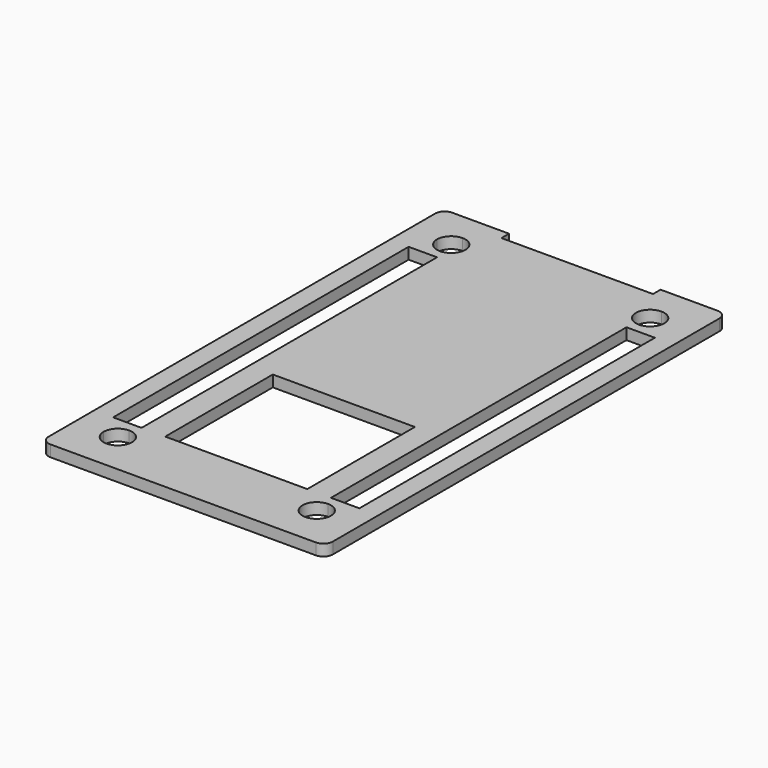
from build123d import *

# Parameters (mm, degrees)
F0_W     = 4
F0_H     = 1
F0_W_2   = 2
F0_H_2   = 39
F0_W_3   = 2.5
F0_H_3   = 0.8
F0_W_4   = 7.5
F0_W_5   = 0.5
F1_DEPTH = 1.2


with BuildPart() as f1:
    # F0 (on Top) → F1 (new body)
    with BuildSketch(Plane.XY):
        with BuildLine():
            Line((-13, 24.5), (-12, 24.5))
            Line((-12, 24.5), (-10.5, 24.5))
            Line((-10.5, 24.5), (-8, 24.5))
            Line((-8, 24.5), (-8, 25.5))
            Line((-8, 25.5), (-8, 26.5))
            Line((-8, 26.5), (-14, 26.5))
            ThreePointArc((-14, 26.5), (-14.7071067812, 26.2071067812), (-15, 25.5))
            Line((-15, 25.5), (-15, 19.5))
            Line((-15, 19.5), (-13, 19.5))
            Line((-13, 19.5), (-13, 22))
            Line((-13, 22), (-13, 23.5))
            Line((-13, 23.5), (-13, 24.5))
        make_face()
        with BuildLine():
            Line((-10.5, 24.5), (-12, 24.5))
            ThreePointArc((-12, 24.5), (-12.7071067812, 24.2071067812), (-13, 23.5))
            Line((-13, 23.5), (-13, 22))
            Line((-13, 22), (-12, 22))
            ThreePointArc((-12, 22), (-11.5606601718, 23.0606601718), (-10.5, 23.5))
            Line((-10.5, 23.5), (-10.5, 24.5))
        make_face()
        with BuildLine():
            ThreePointArc((-13, 23.5), (-12.7071067812, 24.2071067812), (-12, 24.5))
            Line((-12, 24.5), (-13, 24.5))
            Line((-13, 24.5), (-13, 23.5))
        make_face()
        with BuildLine():
            Line((-8, 24.5), (-10.5, 24.5))
            Line((-10.5, 24.5), (-10.5, 23.5))
            ThreePointArc((-10.5, 23.5), (-9.4393398282, 23.0606601718), (-9, 22))
            ThreePointArc((-9, 22), (-9.4393398282, 20.9393398282), (-10.5, 20.5))
            Line((-10.5, 20.5), (-10.5, 19.5))
            Line((-10.5, 19.5), (-10, 19.5))
            Line((-10, 19.5), (10, 19.5))
            Line((10, 19.5), (10.5, 19.5))
            Line((10.5, 19.5), (10.5, 20.5))
            ThreePointArc((10.5, 20.5), (9, 22), (10.5, 23.5))
            Line((10.5, 23.5), (10.5, 24.5))
            Line((10.5, 24.5), (8, 24.5))
            Line((8, 24.5), (4, 24.5))
            Line((4, 24.5), (4, 20))
            Line((4, 20), (-4, 20))
            Line((-4, 20), (-4, 24.5))
            Line((-4, 24.5), (-8, 24.5))
        make_face()
        with Locations((-6, 25)):
            Rectangle(F0_W, F0_H)
        with BuildLine():
            Line((-12, 22), (-13, 22))
            Line((-13, 22), (-13, 19.5))
            Line((-13, 19.5), (-10.5, 19.5))
            Line((-10.5, 19.5), (-10.5, 20.5))
            ThreePointArc((-10.5, 20.5), (-11.5606601718, 20.9393398282), (-12, 22))
        make_face()
        with Locations((-2, 25)):
            Rectangle(F0_W, F0_H)
        Polygon((0, 24.5), (-4, 24.5), (-4, 20), (4, 20), (4, 24.5), align=None)
        with Locations((-14, 0)):
            Rectangle(F0_W_2, F0_H_2)
        with Locations((2, 25)):
            Rectangle(F0_W, F0_H)
        with Locations((-11.75, -19.9)):
            Rectangle(F0_W_3, F0_H_3)
        with Locations((-14, -19.9)):
            Rectangle(F0_W_2, F0_H_3)
        with Locations((6, 25)):
            Rectangle(F0_W, F0_H)
        with BuildLine():
            Line((-10.5, -20.3), (-13, -20.3))
            Line((-13, -20.3), (-13, -22))
            Line((-13, -22), (-12, -22))
            ThreePointArc((-12, -22), (-11.5606601718, -20.9393398282), (-10.5, -20.5))
            Line((-10.5, -20.5), (-10.5, -20.3))
        make_face()
        with BuildLine():
            Line((-13, -22), (-13, -20.3))
            Line((-13, -20.3), (-15, -20.3))
            Line((-15, -20.3), (-15, -25.5))
            ThreePointArc((-15, -25.5), (-14.7071067812, -26.2071067812), (-14, -26.5))
            Line((-14, -26.5), (14, -26.5))
            ThreePointArc((14, -26.5), (14.7071067812, -26.2071067812), (15, -25.5))
            Line((15, -25.5), (15, -20.3))
            Line((15, -20.3), (13, -20.3))
            Line((13, -20.3), (13, -22))
            Line((13, -22), (13, -23.5))
            ThreePointArc((13, -23.5), (12.7071067812, -24.2071067812), (12, -24.5))
            Line((12, -24.5), (10.5, -24.5))
            Line((10.5, -24.5), (-10.5, -24.5))
            Line((-10.5, -24.5), (-12, -24.5))
            ThreePointArc((-12, -24.5), (-12.7071067812, -24.2071067812), (-13, -23.5))
            Line((-13, -23.5), (-13, -22))
        make_face()
        Polygon((-10, -19.5), (-10.5, -19.5), (-10.5, -20.3), (-7.5, -20.3), (-7.5, -19.5), align=None)
        Polygon((10, 19.5), (-10, 19.5), (-10, -19.5), (-7.5, -19.5), (-7.5, -5.3), (7.5, -5.3), (7.5, -19.5), (10, -19.5), (10, 19.1765315831), align=None)
        with BuildLine():
            Line((8, 25.5), (8, 24.5))
            Line((8, 24.5), (10.5, 24.5))
            Line((10.5, 24.5), (12, 24.5))
            ThreePointArc((12, 24.5), (12.7071067812, 24.2071067812), (13, 23.5))
            Line((13, 23.5), (13, 22))
            Line((13, 22), (13, 19.5))
            Line((13, 19.5), (15, 19.5))
            Line((15, 19.5), (15, 25.5))
            ThreePointArc((15, 25.5), (14.7071067812, 26.2071067812), (14, 26.5))
            Line((14, 26.5), (8, 26.5))
            Line((8, 26.5), (8, 25.5))
        make_face()
        with BuildLine():
            Line((-12, -22), (-13, -22))
            Line((-13, -22), (-13, -23.5))
            ThreePointArc((-13, -23.5), (-12.7071067812, -24.2071067812), (-12, -24.5))
            Line((-12, -24.5), (-10.5, -24.5))
            Line((-10.5, -24.5), (-10.5, -23.5))
            ThreePointArc((-10.5, -23.5), (-11.5606601718, -23.0606601718), (-12, -22))
        make_face()
        with BuildLine():
            Line((-7.5, -20.3), (-10.5, -20.3))
            Line((-10.5, -20.3), (-10.5, -20.5))
            ThreePointArc((-10.5, -20.5), (-9.4393398282, -20.9393398282), (-9, -22))
            ThreePointArc((-9, -22), (-9.4393398282, -23.0606601718), (-10.5, -23.5))
            Line((-10.5, -23.5), (-10.5, -24.5))
            Line((-10.5, -24.5), (10.5, -24.5))
            Line((10.5, -24.5), (10.5, -23.5))
            ThreePointArc((10.5, -23.5), (9, -22), (10.5, -20.5))
            Line((10.5, -20.5), (10.5, -20.3))
            Line((10.5, -20.3), (10, -20.3))
            Line((10, -20.3), (7.5, -20.3))
            Line((7.5, -20.3), (0, -20.3))
            Line((0, -20.3), (-7.5, -20.3))
        make_face()
        with BuildLine():
            Line((12, 24.5), (10.5, 24.5))
            Line((10.5, 24.5), (10.5, 23.5))
            ThreePointArc((10.5, 23.5), (11.5606601718, 23.0606601718), (12, 22))
            Line((12, 22), (13, 22))
            Line((13, 22), (13, 23.5))
            ThreePointArc((13, 23.5), (12.7071067812, 24.2071067812), (12, 24.5))
        make_face()
        with Locations((-3.75, -19.9)):
            Rectangle(F0_W_4, F0_H_3)
        with BuildLine():
            Line((10.5, 20.5), (10.5, 19.5))
            Line((10.5, 19.5), (13, 19.5))
            Line((13, 19.5), (13, 22))
            Line((13, 22), (12, 22))
            ThreePointArc((12, 22), (11.5606601718, 20.9393398282), (10.5, 20.5))
        make_face()
        with Locations((3.75, -19.9)):
            Rectangle(F0_W_4, F0_H_3)
        with Locations((8.75, -19.9)):
            Rectangle(F0_W_3, F0_H_3)
        with Locations((10.25, -19.9)):
            Rectangle(F0_W_5, F0_H_3)
        with Locations((14, 0)):
            Rectangle(F0_W_2, F0_H_2)
        with Locations((11.75, -19.9)):
            Rectangle(F0_W_3, F0_H_3)
        with Locations((14, -19.9)):
            Rectangle(F0_W_2, F0_H_3)
        with BuildLine():
            Line((10.5, -23.5), (10.5, -24.5))
            Line((10.5, -24.5), (12, -24.5))
            ThreePointArc((12, -24.5), (12.7071067812, -24.2071067812), (13, -23.5))
            Line((13, -23.5), (13, -22))
            Line((13, -22), (12, -22))
            ThreePointArc((12, -22), (11.5606601718, -23.0606601718), (10.5, -23.5))
        make_face()
        with BuildLine():
            Line((13, -20.3), (10.5, -20.3))
            Line((10.5, -20.3), (10.5, -20.5))
            ThreePointArc((10.5, -20.5), (11.5606601718, -20.9393398282), (12, -22))
            Line((12, -22), (13, -22))
            Line((13, -22), (13, -20.3))
        make_face()
    extrude(amount=F1_DEPTH)


solid = f1.part
